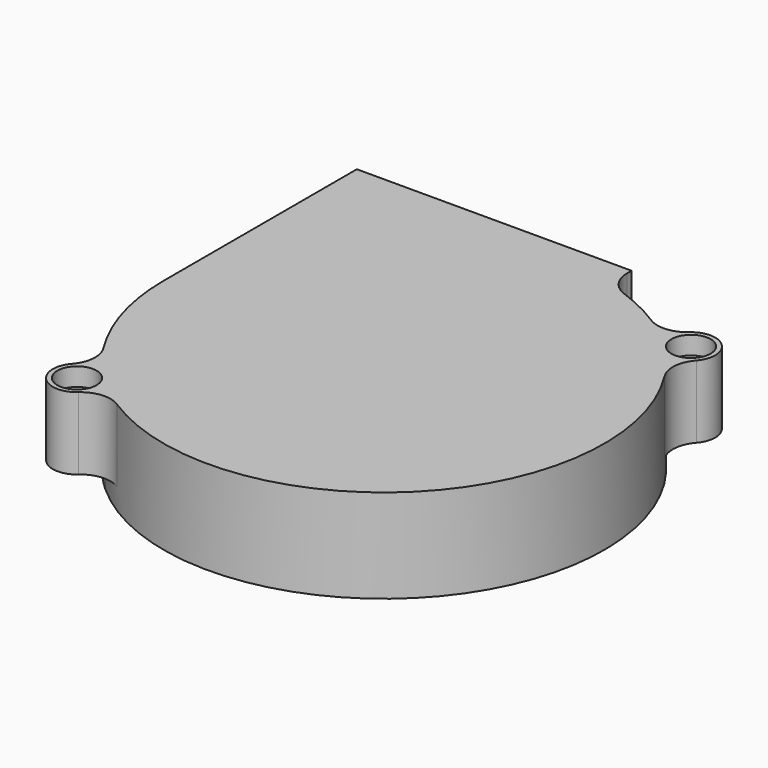
from build123d import *

# Parameters (mm, degrees)
F1_DEPTH       = 15.5
F2_R           = 25
F3_DEPTH       = 3.5
F5_D           = 3.3
F5_CBORE_D     = 6.5
F5_CBORE_DEPTH = 3
F6_T1_DEPTH    = 12
F6_T3_DEPTH    = 15.5


# Not quite as in the source:
# - a fillet or chamfer that OpenCascade refuses, or shapes differently, is made with other operations: its cross-section is extruded or revolved along the edge and cut away or added


with BuildPart() as f1:
    # F0 (on Top) → F1 (new body)
    with BuildSketch(Plane.XY):
        with BuildLine():
            ThreePointArc((27.1408006584, 24.4054694612), (31.0773430331, 31.0773430331), (24.4054694612, 27.1408006584))
            ThreePointArc((24.4054694612, 27.1408006584), (17.2024322308, 32.1920226973), (9, 35.3730123116))
            Line((9, 35.3730123116), (9, 40))
            Line((9, 40), (-36.5, 40))
            Line((-36.5, 40), (-36.5, 0))
            ThreePointArc((-36.5, 0), (-34.0799737678, -13.0692535358), (-27.1408006584, -24.4054694612))
            ThreePointArc((-27.1408006584, -24.4054694612), (-31.0773430331, -31.0773430331), (-24.4054694612, -27.1408006584))
            ThreePointArc((-24.4054694612, -27.1408006584), (25.8093975133, -25.8093975133), (27.1408006584, 24.4054694612))
        make_face()
    extrude(amount=F1_DEPTH)

    # F2 (on face) → F3 (cut)
    with BuildSketch(Plane(origin=(0, 0, 0), x_dir=(1, 0, 0), z_dir=(0, 0, -1))):
        with BuildLine():
            ThreePointArc((-27.1408006584, 24.4054694612), (-25.8093975133, 25.8093975133), (-24.4054694612, 27.1408006584))
            ThreePointArc((-24.4054694612, 27.1408006584), (-31.0773430331, 31.0773430331), (-27.1408006584, 24.4054694612))
        make_face()
        with BuildLine():
            ThreePointArc((27.1408006584, -24.4054694612), (25.8093975133, -25.8093975133), (24.4054694612, -27.1408006584))
            ThreePointArc((24.4054694612, -27.1408006584), (31.0773430331, -31.0773430331), (27.1408006584, -24.4054694612))
        make_face()
        Circle(F2_R)
    extrude(amount=-F3_DEPTH, mode=Mode.SUBTRACT)

    # F5 (through all)
    with Locations(Plane.XY.offset(15.5)):
        with Locations((-28.2489159084, -28.2489159084), (28.2489159084, 28.2489159084)):
            CounterBoreHole(F5_D / 2, F5_CBORE_D / 2, F5_CBORE_DEPTH)

    # F6: fillet of radius 5 on 5 edges, made by hand

    # F6_s2 → F6_t1 (join)
    with BuildSketch(Plane.XY.offset(3.5)):
        with BuildLine():
            ThreePointArc((-30.783749931, -19.6114951033), (-30.0157488678, -22.6856125629), (-31.2497097164, -25.6040649633))
            ThreePointArc((-31.2497097164, -25.6040649633), (-29.369056893, -24.4089570317), (-27.1408006584, -24.4054694612))
            ThreePointArc((-27.1408006584, -24.4054694612), (-29.0612962165, -22.0837284492), (-30.783749931, -19.6114951033))
        make_face()
        with BuildLine():
            ThreePointArc((-19.6114951033, -30.783749931), (-22.6856125629, -30.0157488678), (-25.6040649633, -31.2497097164))
            ThreePointArc((-25.6040649633, -31.2497097164), (-24.4089570317, -29.369056893), (-24.4054694612, -27.1408006584))
            ThreePointArc((-24.4054694612, -27.1408006584), (-22.0837284492, -29.0612962165), (-19.6114951033, -30.783749931))
        make_face()
        with BuildLine():
            ThreePointArc((30.783749931, 19.6114951033), (30.0157488678, 22.6856125629), (31.2497097164, 25.6040649633))
            ThreePointArc((31.2497097164, 25.6040649633), (29.369056893, 24.4089570317), (27.1408006584, 24.4054694612))
            ThreePointArc((27.1408006584, 24.4054694612), (29.0612962165, 22.0837284492), (30.783749931, 19.6114951033))
        make_face()
        with BuildLine():
            ThreePointArc((19.6114951033, 30.783749931), (22.6856125629, 30.0157488678), (25.6040649633, 31.2497097164))
            ThreePointArc((25.6040649633, 31.2497097164), (24.4089570317, 29.369056893), (24.4054694612, 27.1408006584))
            ThreePointArc((24.4054694612, 27.1408006584), (22.0837284492, 29.0612962165), (19.6114951033, 30.783749931))
        make_face()
    extrude(amount=F6_T1_DEPTH)

    # F6_s4 → F6_t3 (join)
    with BuildSketch(Plane.XY):
        with BuildLine():
            ThreePointArc((12.313253012, 34.3603521557), (9.9113734005, 36.189206534), (9, 39.0672497112))
            Line((9, 39.0672497112), (9, 35.3730123116))
            ThreePointArc((9, 35.3730123116), (10.6686483978, 34.9060158334), (12.313253012, 34.3603521557))
        make_face()
    extrude(amount=F6_T3_DEPTH)


solid = f1.part
